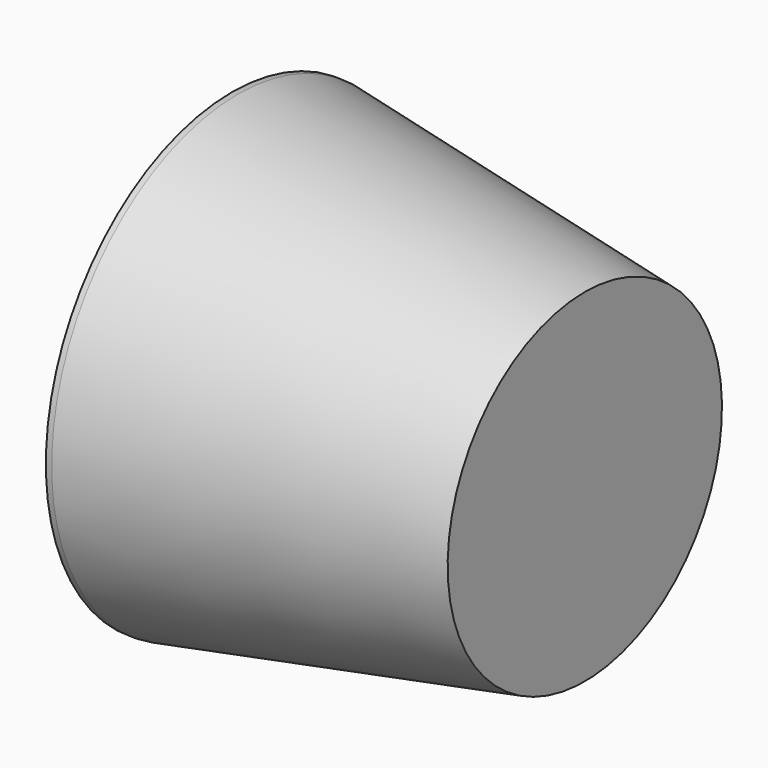
from build123d import *

# Parameters (mm, degrees)
F2_R     = 38
F3_DEPTH = 95


with BuildPart() as f1:
    # F0 (on Front) → F1 (revolve)
    with BuildSketch(Plane.XZ):
        with BuildLine():
            Line((5.073e-07, 40.0000000001), (-1e-10, 0))
            Line((0, 0), (7.5000005075, -7e-10))
            Line((7.5000005075, -7e-10), (7.5000005075, 42.0000000001))
            ThreePointArc((7.5000005075, 42.0000000001), (6.9142140698, 40.5857864377), (5.5000005075, 40.0000000001))
            Line((5.5000005075, 40.0000000001), (5.073e-07, 40.0000000001))
        make_face()
        Polygon((7.5000005075, 42.0000000001), (7.5000005075, -7e-10), (9.0000005075, -9e-10), (9.0000005075, 59.9999999993), (7.5000005075, 59.9999999993), align=None)
        Polygon((9.0000005075, 59.9999999993), (9.0000005075, -9e-10), (98.5000005577, -9.5e-09), (98.5000005577, 43.954244746), (98.5000005577, 44.218735217), align=None)
    revolve(axis=Axis((46.8394961208, 0, 0), (1, 0, 0)))

    # F2 (on face) → F3 (cut)
    with BuildSketch(Plane(origin=(2.536e-07, 0, 0), x_dir=(0, -1, 0), z_dir=(-1, 0, 0))):
        Circle(F2_R)
    extrude(amount=-F3_DEPTH, mode=Mode.SUBTRACT)


solid = f1.part
